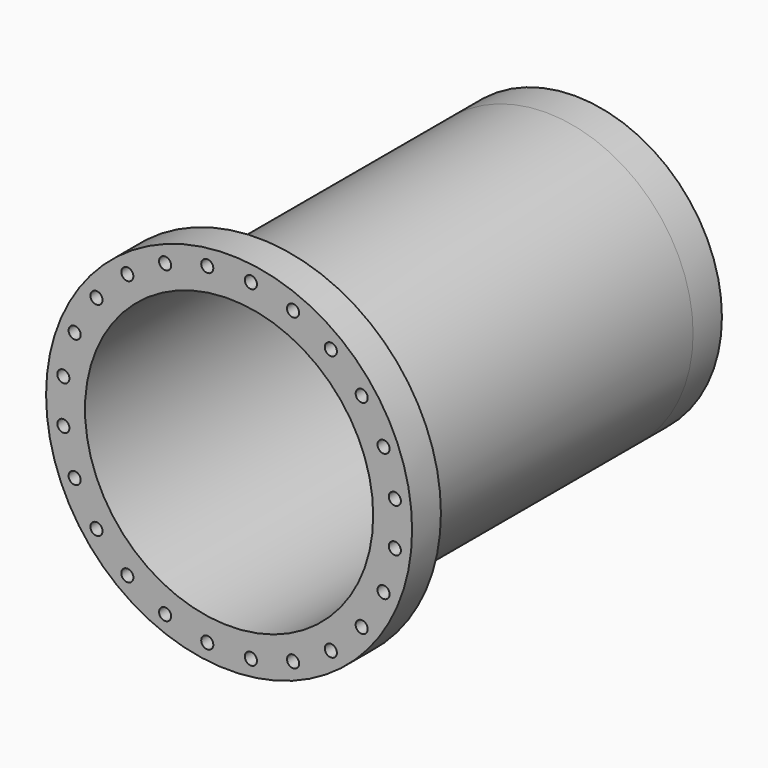
from build123d import *

# Parameters (mm, degrees)
F0_R      = 102
F0_R_2    = 100
F1_DEPTH  = 250
F2_R      = 127
F2_R_2    = 102
F2_R_3    = 100
F3_DEPTH  = 25
F4_R      = 102
F4_R_2    = 100
F5_DEPTH  = 25
F7_D      = 8.4
F8_R      = 50
F9_DEPTH  = 300.001
F10_D     = 8.4
F10_DEPTH = 9
F10_TIP   = 2.5236145999


with BuildPart() as f1:
    # F0 (on Front) → F1 (new body)
    with BuildSketch(Plane.XZ):
        Circle(F0_R)
        Circle(F0_R_2, mode=Mode.SUBTRACT)
    extrude(amount=F1_DEPTH)

    # F2 (on face) → F3 (join)
    with BuildSketch(Plane.XZ.offset(250)):
        Circle(F2_R)
        Circle(F2_R_2, mode=Mode.SUBTRACT)
        Circle(F2_R_2)
        Circle(F2_R_3, mode=Mode.SUBTRACT)
    extrude(amount=F3_DEPTH)

    # F4 (on face) → F5 (join)
    with BuildSketch(Plane(origin=(0, 0, 0), x_dir=(-1, 0, 0), z_dir=(0, 1, 0))):
        Circle(F4_R)
        Circle(F4_R_2, mode=Mode.SUBTRACT)
        Circle(F4_R_2)
    extrude(amount=F5_DEPTH)

    # F7 (through all)
    with Locations(Plane.XZ.offset(275)):
        with Locations((15.1410382975, 115.0076039194), (44.3912781544, 107.1700257713), (70.616325765, 92.0289874738), (92.0289874738, 70.616325765), (107.1700257713, 44.3912781544), (115.0076039194, 15.1410382975), (115.0076039194, -15.1410382975), (107.1700257713, -44.3912781544), (92.0289874738, -70.616325765), (70.616325765, -92.0289874738), (44.3912781544, -107.1700257713), (15.1410382975, -115.0076039194), (-15.1410382975, -115.0076039194), (-44.3912781544, -107.1700257713), (-70.616325765, -92.0289874738), (-92.0289874738, -70.616325765), (-107.1700257713, -44.3912781544), (-115.0076039194, -15.1410382975), (-115.0076039194, 15.1410382975), (-107.1700257713, 44.3912781544), (-92.0289874738, 70.616325765), (-70.616325765, 92.0289874738), (-44.3912781544, 107.1700257713), (-15.1410382975, 115.0076039194)):
            Hole(F7_D / 2)

    # F8 (on face) → F9 (cut, through all)
    with BuildSketch(Plane(origin=(0, 25, 0), x_dir=(-1, 0, 0), z_dir=(0, 1, 0))):
        with Locations((-5, 22.5)):
            Circle(F8_R)
    extrude(amount=-F9_DEPTH, mode=Mode.SUBTRACT)

    # F10
    with Locations(Plane(origin=(0, 25, 0), x_dir=(-1, 0, 0), z_dir=(0, 1, 0))):
        with Locations((-5, 87.5), (-29.8744231037, -37.5521696132), (-50.9619407771, -23.4619407771), (-65.0521696132, -2.3744231037), (-70, 22.5), (-65.0521696132, 47.3744231037), (-50.9619407771, 68.4619407771), (-29.8744231037, 82.5521696132), (19.8744231037, 82.5521696132), (40.9619407771, 68.4619407771), (55.0521696132, 47.3744231037), (60, 22.5), (55.0521696132, -2.3744231037), (40.9619407771, -23.4619407771), (19.8744231037, -37.5521696132), (-5, -42.5)):
            Hole(F10_D / 2, depth=F10_DEPTH)
            with Locations((0, 0, -(F10_DEPTH + F10_TIP / 2))):  # 118° drill point
                Cone(0, F10_D / 2, F10_TIP, mode=Mode.SUBTRACT)


solid = f1.part
